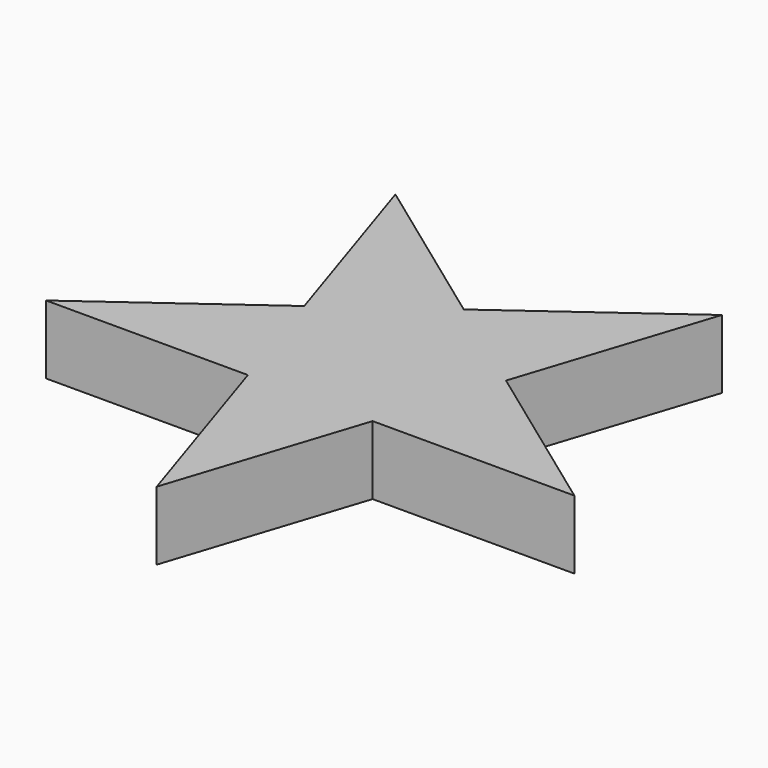
from build123d import *

# Parameters (mm, degrees)
F1_DEPTH = 2


# Not quite as in the source:
# - a feature names something its author has since deleted; it is built from what else it names


with BuildPart() as f1:
    # F0 (on Top) → F1 (new body)
    with BuildSketch(Plane.XY):
        Polygon((-2.9389262615, 0.9549150281), (0, 3.0901699437), (-4.7552825815, 6.5450849719), align=None)
        Polygon((4.7552825815, 6.5450849719), (0, 3.0901699437), (2.9389262615, 0.9549150281), align=None)
        Polygon((2.9389262615, 0.9549150281), (0, 3.0901699437), (-2.9389262615, 0.9549150281), (-1.81635632, -2.5), (1.81635632, -2.5), (2.3776412907, -0.7725424859), align=None)
        Polygon((-1.81635632, -2.5), (-2.9389262615, 0.9549150281), (-7.6942088429, -2.5), align=None)
        Polygon((7.6942088429, -2.5), (2.9389262615, 0.9549150281), (2.3776412907, -0.7725424859), align=None)
        Polygon((7.6942088429, -2.5), (2.3776412907, -0.7725424859), (1.81635632, -2.5), align=None)
        Polygon((1.81635632, -2.5), (-1.81635632, -2.5), (0, -8.0901699437), align=None)
    extrude(amount=F1_DEPTH)


solid = f1.part
